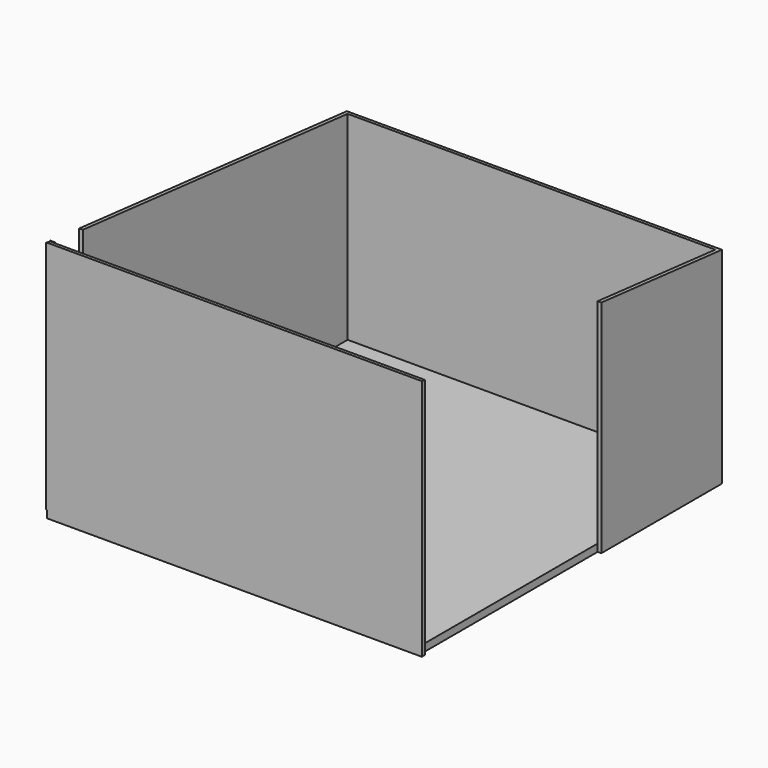
from build123d import *

# Parameters (mm, degrees)
F0_W          = 10200
F0_H          = 10200
F0_W_2        = 10000
F0_H_2        = 10000
F1_DEPTH      = 25
F2_DEPTH      = 6750
F3_W          = 10200
F3_H          = 200
F4_DEPTH      = 10200
F6_DEPTH      = 10200.001
F7_W          = 1000
F7_H          = 2200
F8_DEPTH      = 1400
F8_DEPTH_BACK = 11390
F9_W          = 6000
F9_H          = 6590.1960784314
F10_DEPTH     = 100
F11_TEXT_SIZE = 1216.6990174188
F12_DEPTH     = 25
F14_REACH     = 6597.9908987322


# Not quite as in the source:
# - a feature names something its author has since deleted; it is built from what else it names
# - Text() gives the source's letters only with a copy of the font that has no kerning and outlines rounded to 1/6400 em; it was checked with that copy


with BuildPart() as f1:
    # F0 (on Top) → F1 (new body)
    with BuildSketch(Plane.XY):
        with Locations((5000, 5000)):
            Rectangle(F0_W, F0_H)
        with Locations((5000, 5000)):
            Rectangle(F0_W_2, F0_H_2, mode=Mode.SUBTRACT)
    extrude(amount=F1_DEPTH)

    # F0 (on Top) → F2 (join)
    with BuildSketch(Plane.XY):
        with Locations((5000, 5000)):
            Rectangle(F0_W, F0_H)
        with Locations((5000, 5000)):
            Rectangle(F0_W_2, F0_H_2, mode=Mode.SUBTRACT)
    extrude(amount=F2_DEPTH)

    # F3 (on face) → F4 (join, through all)
    with BuildSketch(Plane.XZ.offset(100)):
        with Locations((5000, -100)):
            Rectangle(F3_W, F3_H)
    extrude(amount=-F4_DEPTH)

    # F5 (on face) → F6 (cut, through all)
    with BuildSketch(Plane.YZ.offset(10100)):
        Polygon((-100, 6400), (10100, 5400), (10100, 6903.0771255493), (-100, 6903.0771255493), align=None)
    extrude(amount=-F6_DEPTH, mode=Mode.SUBTRACT)

    # F7 (on face) → F8 (cut, two sides)
    with BuildSketch(Plane.YZ) as f8_sk:
        with Locations((500, 5290.1960784314)):
            Rectangle(F7_W, F7_H)
    extrude(amount=-F8_DEPTH, mode=Mode.SUBTRACT)
    extrude(f8_sk.sketch, amount=F8_DEPTH_BACK, mode=Mode.SUBTRACT)

    # F9 (on face) → F10 (cut, through all)
    with BuildSketch(Plane.YZ.offset(10100)):
        with Locations((3000, 3095.0980392157)):
            Rectangle(F9_W, F9_H)
    extrude(amount=-F10_DEPTH, mode=Mode.SUBTRACT)

    # F11 (on face) → F12 (join)
    with BuildSketch(Plane(origin=(0, 0, 0), x_dir=(-1, 0, 0), z_dir=(0, 1, 0))):
        with Locations((-7386.3310813904, 1671.2728738785)):
            Text('Atelier 2', F11_TEXT_SIZE, font='Open Sans', text_align=(TextAlign.LEFT, TextAlign.BOTTOM))
    extrude(amount=F12_DEPTH)

    f14_end = Plane(origin=(5000, -50, 6395.0980392157), x_dir=(0, 0.9952285251, -0.097571424), z_dir=(0, 0.097571424, 0.9952285251))
    # F13 (on face) → F14 (join, up to a plane its end follows)
    with BuildSketch(Plane.XY):
        Polygon((-50, 40), (-120, 40), (-120, 30), (-55, 30), (-55, -90), (-120, -90), (-120, -100), (-50, -100), (20, -100), (20, -90), (-45, -90), (-45, 30), (20, 30), (20, 40), align=None)
    f14_long = extrude(amount=F14_REACH, mode=Mode.PRIVATE)
    add(split(f14_long, bisect_by=f14_end, keep=Keep.BOTTOM, mode=Mode.PRIVATE))


solid = f1.part
